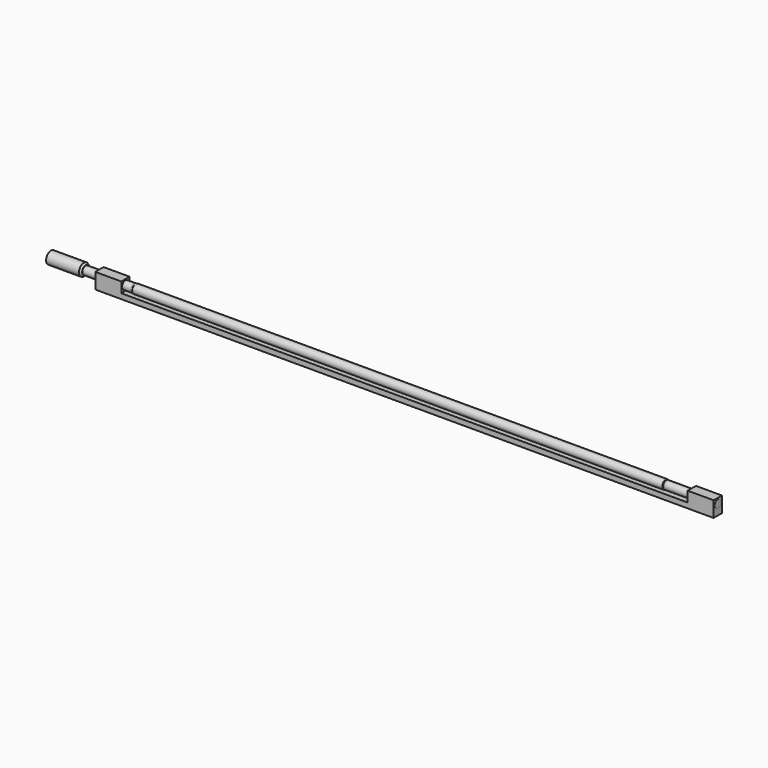
from build123d import *

# Parameters (mm, degrees)
F0_W            = 357
F0_H            = 3
F1_DEPTH        = 3
F2_W            = 6
F2_H            = 6
F3_DEPTH        = 15
F4_W            = 6
F4_H            = 6
F5_DEPTH        = 15
F6_R            = 2.36
F7_DEPTH        = 14
F8_R            = 2.565
F9_DEPTH        = 308
F10_R           = 2.36
F11_DEPTH       = 28
F12_DEPTH       = 15.1
F13_R           = 3.5
F14_DEPTH       = 20
F15_2_S5_R      = 2.36
F15_2_T6_DEPTH  = 5
F15_2_S11_R     = 2.36
F15_2_T12_DEPTH = 5
F17_DEPTH       = 5.8
F18_R           = 0.5


# Not quite as in the source:
# - a fillet or chamfer that OpenCascade refuses, or shapes differently, is made with other operations: its cross-section is extruded or revolved along the edge and cut away or added


with BuildPart() as f1:
    # F0 (on Front) → F1 (new body, symmetric)
    with BuildSketch(Plane.XZ):
        with Locations((178.5, 1.5)):
            Rectangle(F0_W, F0_H)
    extrude(amount=F1_DEPTH, both=True)


with BuildPart() as f3:
    # F2 (on face) → F3 (new body)
    with BuildSketch(Plane.YZ.offset(357)):
        with Locations((0, 6)):
            Rectangle(F2_W, F2_H)
    extrude(amount=-F3_DEPTH)



with BuildPart() as f5:
    # F4 (on face) → F5 (new body)
    with BuildSketch(Plane(origin=(0, 0, 0), x_dir=(0, -1, 0), z_dir=(-1, 0, 0))):
        with Locations((0, 6)):
            Rectangle(F4_W, F4_H)
    extrude(amount=-F5_DEPTH)



with BuildPart() as f7:
    # F6 (on face) → F7 (new body)
    with BuildSketch(Plane(origin=(342, 0, 0), x_dir=(0, -1, 0), z_dir=(-1, 0, 0))):
        with Locations((0, 6)):
            Circle(F6_R)
    extrude(amount=F7_DEPTH)

    # F8 (on face) → F9 (join)
    with BuildSketch(Plane(origin=(328, 0, 0), x_dir=(0, -1, 0), z_dir=(-1, 0, 0))):
        with Locations((0, 6)):
            Circle(F8_R)
    extrude(amount=F9_DEPTH)


with BuildPart() as f5_1:
    add(f5.part)

    add(f7.part)  # F11 merges F7
    # F10 (on face) → F11 (join)
    with BuildSketch(Plane(origin=(20, 0, 0), x_dir=(0, -1, 0), z_dir=(-1, 0, 0))):
        with Locations((0, 6)):
            Circle(F10_R)
    extrude(amount=F11_DEPTH)


with BuildPart() as f3_1:
    add(f3.part)

    add(f5_1.part)  # F12 merges F5
    # F6 (on face) → F12 (join)
    with BuildSketch(Plane(origin=(342, 0, 0), x_dir=(0, -1, 0), z_dir=(-1, 0, 0))):
        with Locations((0, 6)):
            Circle(F6_R)
    extrude(amount=-F12_DEPTH)

    # F15#2: chamfer of 1 on 2 edges, made by hand


with BuildPart() as f14:
    # F13 (on face) → F14 (new body)
    with BuildSketch(Plane(origin=(-8, 0, 0), x_dir=(0, -1, 0), z_dir=(-1, 0, 0))):
        with Locations((0, 6)):
            Circle(F13_R)
    extrude(amount=F14_DEPTH)

    # F15: chamfer of 1 on 1 edges, made by hand

    # F15_s1 → F15_t2 (revolve, cut)
    with BuildSketch(Plane.XY.offset(6)):
        Polygon((-9, -3.5), (-8, -2.5), (-8, -3.5), align=None)
    revolve(axis=Axis((-8, 0, 6), (-1, 0, 0)), mode=Mode.SUBTRACT)

    # F16 (on face) → F17 (cut)
    with BuildSketch(Plane(origin=(-28, 0, 0), x_dir=(0, -1, 0), z_dir=(-1, 0, 0))):
        Polygon((0, 3.6905989232), (2, 4.8452994616), (2, 7.1547005384), (0, 8.3094010768), (-2, 7.1547005384), (-2, 4.8452994616), align=None)
    extrude(amount=-F17_DEPTH, mode=Mode.SUBTRACT)

    # F18
    f18_edges = [f14.edges().sort_by_distance(p)[0] for p in [
        (-22.2, 1, 4.267949),
        (-22.2, -1, 4.267949),
        (-22.2, -2, 6),
        (-22.2, -1, 7.732051),
        (-22.2, 1, 7.732051),
        (-22.2, 2, 6),
    ]]
    fillet(f18_edges, radius=F18_R)


with BuildPart() as f15_2_tool2:
    # F15_2_s3 → F15_2_t4 (revolve)
    with BuildSketch(Plane.XY.offset(6)):
        Polygon((21, -2.565), (20, -1.565), (20, -2.565), align=None)
    revolve(axis=Axis((20, 0, 6), (-1, 0, 0)))

    # F15_2_s5 → F15_2_t6 (cut, symmetric)
    with BuildSketch(Plane.YZ.offset(20.5)):
        with Locations((0, 6)):
            Circle(F15_2_S5_R)
    extrude(amount=F15_2_T6_DEPTH, both=True, mode=Mode.SUBTRACT)


with BuildPart() as f3_2:
    add(f3_1.part)

    # F15_2_t1: cut F15_2_tool2
    add(f15_2_tool2.part, mode=Mode.SUBTRACT)


with BuildPart() as f15_2_tool8:
    # F15_2_s9 → F15_2_t10 (revolve)
    with BuildSketch(Plane.XY.offset(6)):
        Polygon((328, -1.565), (327, -2.565), (328, -2.565), align=None)
    revolve(axis=Axis((328, 0, 6), (-1, 0, 0)))

    # F15_2_s11 → F15_2_t12 (cut, symmetric)
    with BuildSketch(Plane.YZ.offset(327.5)):
        with Locations((0, 6)):
            Circle(F15_2_S11_R)
    extrude(amount=F15_2_T12_DEPTH, both=True, mode=Mode.SUBTRACT)


with BuildPart() as f3_3:
    add(f3_2.part)

    # F15_2_t7: cut F15_2_tool8
    add(f15_2_tool8.part, mode=Mode.SUBTRACT)


with BuildPart() as f1_1:
    add(f1.part)

    # F19: union F3, F14
    add(f3_3.part)
    add(f14.part)


solid = f1_1.part
